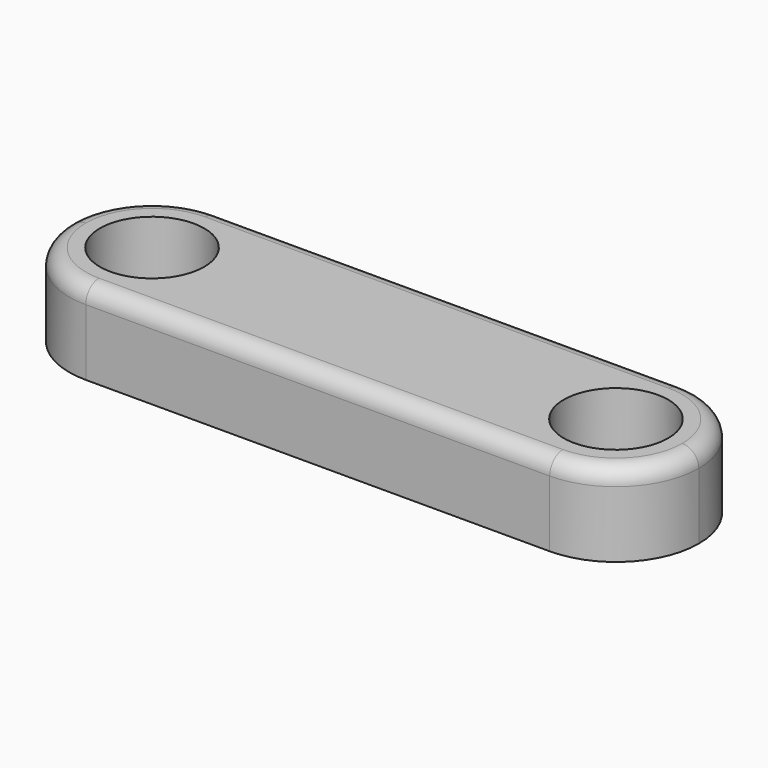
from build123d import *

# Parameters (mm, degrees)
F0_R     = 3.15
F1_DEPTH = 5
F2_R     = 4.99999
F3_R     = 1


# Not quite as in the source:
# - a fillet or chamfer is up to 0.001 mm smaller than in the source, because OpenCascade refuses the exact size


with BuildPart() as f1:
    # F0 (on Top) → F1 (new body)
    with BuildSketch(Plane.XY):
        Polygon((-49.8123717308, 43.8505291194), (-54.8123717308, 43.8505291194), (-54.8123717308, 33.8505291194), (-16.8123717308, 33.8505291194), (-16.8123717308, 43.8505291194), align=None)
        with Locations((-49.8123717308, 38.8505291194)):
            Circle(F0_R, mode=Mode.SUBTRACT)
        with Locations((-21.8123717308, 38.8505291194)):
            Circle(F0_R, mode=Mode.SUBTRACT)
    extrude(amount=F1_DEPTH)

    # F2 (radius 5 in the source; OpenCascade refuses exactly that, so slightly less here)
    f2_edges = [f1.edges().sort_by_distance(p)[0] for p in [
        (-54.812372, 33.850529, 2.5),
        (-54.812372, 43.850529, 2.5),
        (-16.812372, 43.850529, 2.5),
        (-16.812372, 33.850529, 2.5),
    ]]
    fillet(f2_edges, radius=F2_R)

    # F3
    f3_edges = [f1.edges().sort_by_distance(p)[0] for p in [
        (-35.812372, 33.850529, 5),
        (-35.812372, 43.850529, 5),
    ]]
    fillet(f3_edges, radius=F3_R)


solid = f1.part
